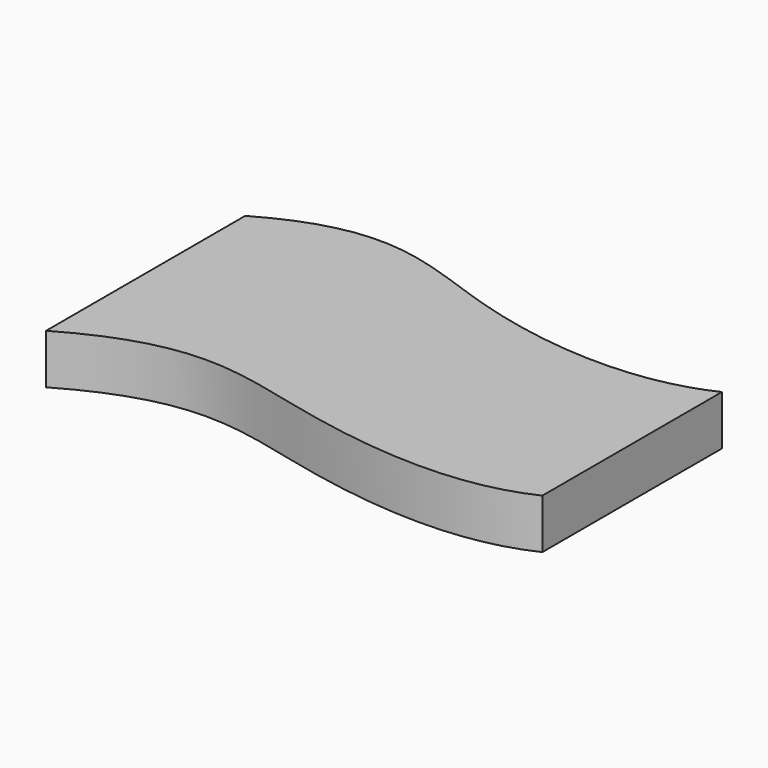
from build123d import *

# Parameters (mm, degrees)
F1_DEPTH = 7.62


with BuildPart() as f1:
    # F0 (on Top) → F1 (new body)
    with BuildSketch(Plane.XY):
        with BuildLine():
            add(Edge.make_bspline(
                [(-36.4998, 19.05), (-20.3205329989, 28.3664337277), (-2.8404673129, 16.9025570855), (26.0014676247, 14.0284521013), (36.4998, 19.05)],
                knots=[0, 0, 0, 0, 0.5, 1, 1, 1, 1], degree=3))
            Line((-36.4998, 19.05), (-36.4998, -19.05))
            add(Edge.make_bspline(
                [(-36.4998, -19.05), (-20.3057624329, -9.7250610044), (-2.8949336053, -16.7114442079), (26.0110518853, -20.3326853111), (36.4998, -15.3157217428)],
                knots=[0, 0, 0, 0, 0.5004564659, 1, 1, 1, 1], degree=3))
            Line((36.4998, -15.3157217428), (36.4998, 19.05))
        make_face()
    extrude(amount=F1_DEPTH)


solid = f1.part
